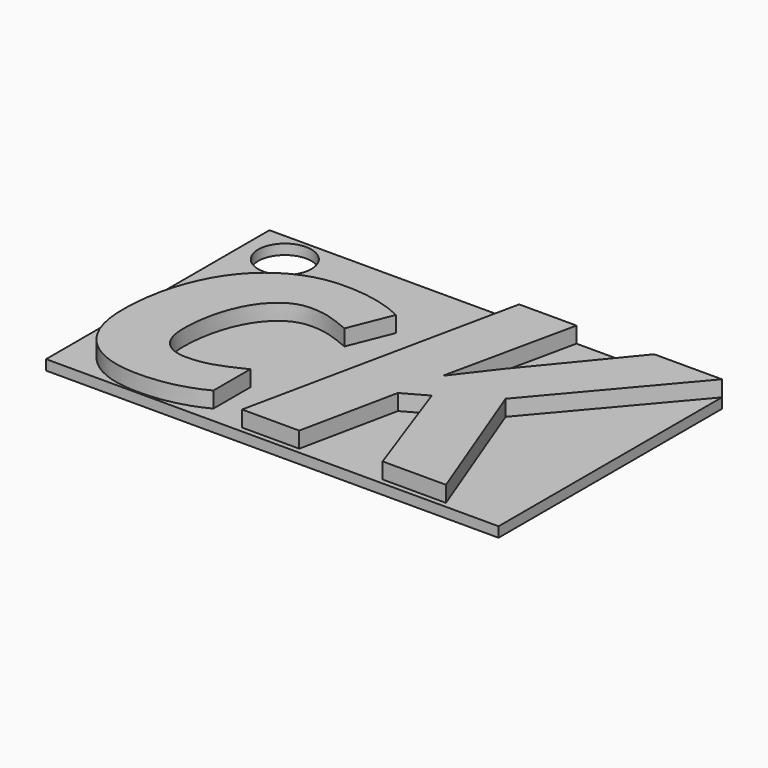
from build123d import *

# Parameters (mm, degrees)
F0_TEXT_SIZE = 67.3100028911
F1_DEPTH     = 2.794
F2_R         = 4.6625417774
F3_DEPTH     = 1.778


# Not quite as in the source:
# - Text() gives the source's letters only with a copy of the font that has no kerning and outlines rounded to 1/6400 em; it was checked with that copy


with BuildPart() as f1:
    # F0 (on Top) → F1 (new body)
    with BuildSketch(Plane.XY):
        with Locations((-24.7046593577, -33.9534860104)):
            Text('cK', F0_TEXT_SIZE, font='Open Sans', font_style=FontStyle.BOLDITALIC, text_align=(TextAlign.LEFT, TextAlign.BOTTOM))
    extrude(amount=F1_DEPTH)


with BuildPart() as f3:
    # F2 (on face) → F3 (new body)
    with BuildSketch(Plane(origin=(0, 0, 0), x_dir=(1, 0, 0), z_dir=(0, 0, -1))):
        Polygon((55.2680378274, 34.8678845912), (-24.0950603038, 34.8678845912), (-24.0950603038, -14.0995457411), (55.2680378274, -14.0995457411), (55.2680378274, 27.6395026594), (55.2680378274, 30.7964943349), (55.2680378274, 33.9534860104), align=None)
        with Locations((-17.0687995851, -8.686799556)):
            Circle(F2_R, mode=Mode.SUBTRACT)
    extrude(amount=F3_DEPTH)


solid = Compound([f1.part, f3.part])
